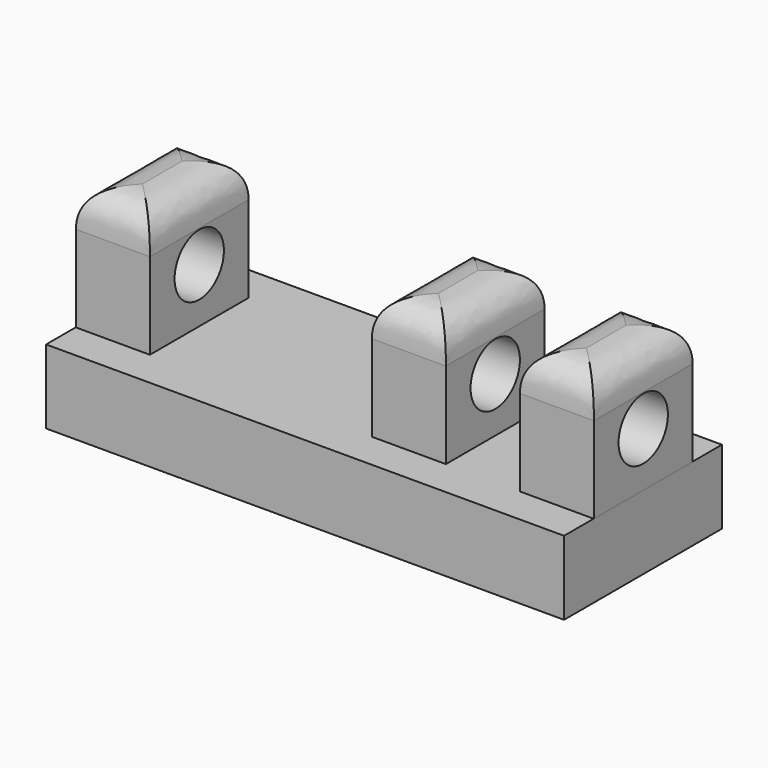
from build123d import *

# Parameters (mm, degrees)
F0_W        = 3
F0_H        = 5
F1_DEPTH    = 5
F2_T1_DEPTH = 12.5
F2_T3_DEPTH = 10.5
F3_R        = 1.25
F4_DEPTH    = 3.03
F0_W_2      = 21
F0_H_2      = 7.9999981078
F9_DEPTH    = 3


# Not quite as in the source:
# - a fillet or chamfer that OpenCascade refuses, or shapes differently, is made with other operations: its cross-section is extruded or revolved along the edge and cut away or added


with BuildPart() as f1:
    # F0 (on Top) → F1 (new body)
    with BuildSketch(Plane.XY):
        with Locations((-56.206721127, 50.7836565375)):
            Rectangle(F0_W, F0_H)
    extrude(amount=F1_DEPTH)

    # F2: fillet of radius 1.5 on 4 edges, made by hand

    # F2_s2 → F2_t1 (cut)
    with BuildSketch(Plane.XZ.offset(-57.0336565375)):
        with BuildLine():
            add(Edge.make_bspline(
                [(-54.706721127, 3.5), (-54.706721127, 5), (-56.206721127, 5)],
                knots=[0, 0, 0, 1, 1, 1], degree=2, weights=[1, 1, 1]))
            Line((-56.206721127, 5), (-54.706721127, 5))
            Line((-54.706721127, 5), (-54.706721127, 3.5))
        make_face()
        with BuildLine():
            add(Edge.make_bspline(
                [(-57.706721127, 3.5), (-57.706721127, 5), (-56.206721127, 5)],
                knots=[0, 0, 0, 1, 1, 1], degree=2, weights=[1, 1, 1]))
            Line((-56.206721127, 5), (-57.706721127, 5))
            Line((-57.706721127, 5), (-57.706721127, 3.5))
        make_face()
    extrude(amount=F2_T1_DEPTH, mode=Mode.SUBTRACT)

    # F2_s4 → F2_t3 (cut)
    with BuildSketch(Plane.YZ.offset(-61.456721127)):
        with BuildLine():
            add(Edge.make_bspline(
                [(53.2836565375, 3.5), (53.2836565375, 5), (51.7836565375, 5)],
                knots=[0, 0, 0, 1, 1, 1], degree=2, weights=[1, 1, 1]))
            Line((51.7836565375, 5), (53.2836565375, 5))
            Line((53.2836565375, 5), (53.2836565375, 3.5))
        make_face()
        with BuildLine():
            add(Edge.make_bspline(
                [(48.2836565375, 3.5), (48.2836565375, 5), (49.7836565375, 5)],
                knots=[0, 0, 0, 1, 1, 1], degree=2, weights=[1, 1, 1]))
            Line((49.7836565375, 5), (48.2836565375, 5))
            Line((48.2836565375, 5), (48.2836565375, 3.5))
        make_face()
    extrude(amount=F2_T3_DEPTH, mode=Mode.SUBTRACT)

    # F3 (on face) → F4 (cut)
    with BuildSketch(Plane(origin=(-57.706721127, 0, 0), x_dir=(0, -1, 0), z_dir=(-1, 0, 0))):
        with Locations((-50.7836565375, 2.1999999881)):
            Circle(F3_R)
    extrude(amount=-F4_DEPTH, mode=Mode.SUBTRACT)


with BuildPart() as f5_1:
    # F5: copy of F1
    add(f1.part.moved(Location((6, 0, 0))))


with BuildPart() as f6_1:
    # F6: copy of F5_1
    add(f5_1.part.moved(Location((-3, 0, 0))))


with BuildPart() as f6_1_1:
    # F7: moved
    add(f6_1.part.moved(Location((-15, 0, 0))))


with BuildPart() as f1_1:
    # F8: moved
    add(f1.part.moved(Location((0, 0, 3))))


with BuildPart() as f5_1_1:
    # F8: moved
    add(f5_1.part.moved(Location((0, 0, 3))))


with BuildPart() as f6_1_2:
    # F8: moved
    add(f6_1_1.part.moved(Location((0, 0, 3))))


with BuildPart() as f9:
    # F0 (on Top) → F9 (new body)
    with BuildSketch(Plane.XY):
        with Locations((-59.216706872, 50.7836549358)):
            Rectangle(F0_W_2, F0_H_2)
        with Locations((-56.206721127, 50.7836565375)):
            Rectangle(F0_W, F0_H, mode=Mode.SUBTRACT)
        with Locations((-56.206721127, 50.7836565375)):
            Rectangle(F0_W, F0_H)
    extrude(amount=F9_DEPTH)


solid = Compound([f1_1.part, f5_1_1.part, f6_1_2.part, f9.part])
